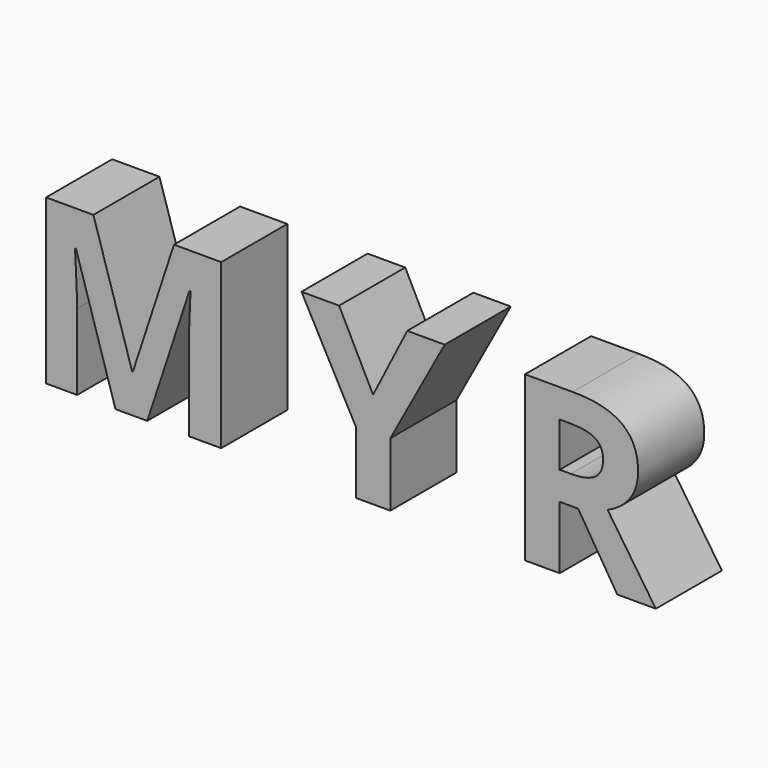
from build123d import *

# Parameters (mm, degrees)
F0_TEXT_SIZE = 70.5555555556
F1_DEPTH     = 25.4


# Not quite as in the source:
# - Text() gives the source's letters only with a copy of the font that has no kerning and outlines rounded to 1/6400 em; it was checked with that copy


with BuildPart() as f1:
    # F0 (on Front) → F1 (new body)
    with BuildSketch(Plane.XZ):
        with Locations((-77.5626046025, -25.8261738985)):
            Text('M Y R', F0_TEXT_SIZE, font='Open Sans', font_style=FontStyle.BOLD, text_align=(TextAlign.LEFT, TextAlign.BOTTOM))
    extrude(amount=F1_DEPTH)


solid = f1.part
